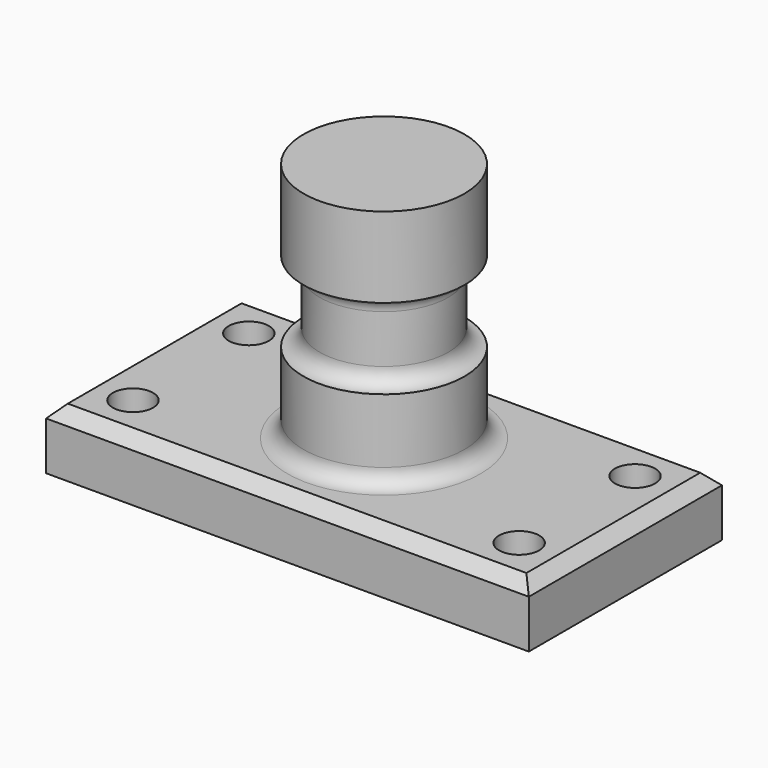
from build123d import *

# Parameters (mm, degrees)
F0_W     = 152.4
F0_H     = 76.2
F1_DEPTH = 19.05
F2_R     = 6.35
F3_DEPTH = 19.05
F4_SIZE  = 3.81
F7_R     = 25.4
F8_DEPTH = 25.4
F9_R     = 5.07999


# Not quite as in the source:
# - a fillet or chamfer is up to 0.001 mm smaller than in the source, because OpenCascade refuses the exact size


with BuildPart() as f1:
    # F0 (on Top) → F1 (new body)
    with BuildSketch(Plane.XY):
        Rectangle(F0_W, F0_H)
    extrude(amount=F1_DEPTH)

    # F2 (on face) → F3 (cut, through all)
    with BuildSketch(Plane.XY.offset(19.05)):
        with Locations((-60.96, 22.86)):
            Circle(F2_R)
        with Locations((-60.96, -22.86)):
            Circle(F2_R)
        with Locations((60.96, 22.86)):
            Circle(F2_R)
        with Locations((60.96, -22.86)):
            Circle(F2_R)
    extrude(amount=-F3_DEPTH, mode=Mode.SUBTRACT)

    # F4
    f4_edges = [f1.edges().sort_by_distance(p)[0] for p in [
        (0, -38.1, 19.05),
        (76.2, 0, 19.05),
        (0, 38.1, 19.05),
        (-76.2, 0, 19.05),
    ]]
    chamfer(f4_edges, length=F4_SIZE)

    # F5 (on Front) → F6 (revolve)
    with BuildSketch(Plane.XZ):
        Polygon((0, 69.85), (0, 19.05), (25.4, 19.05), (25.4, 44.45), (20.32, 44.45), (20.32, 69.85), align=None)
    revolve(axis=Axis((0, 0, 44.45), (0, 0, 1)))

    # F7 (on face) → F8 (join)
    with BuildSketch(Plane.XY.offset(69.85)):
        Circle(F7_R)
    extrude(amount=F8_DEPTH)

    # F9 (radius 5.08 in the source; OpenCascade refuses exactly that, so slightly less here)
    f9_edges = [f1.edges().sort_by_distance(p)[0] for p in [
        (-25.4, 0, 19.05),
        (-20.32, 0, 44.45),
        (-20.32, 0, 69.85),
    ]]
    fillet(f9_edges, radius=F9_R)


solid = f1.part
